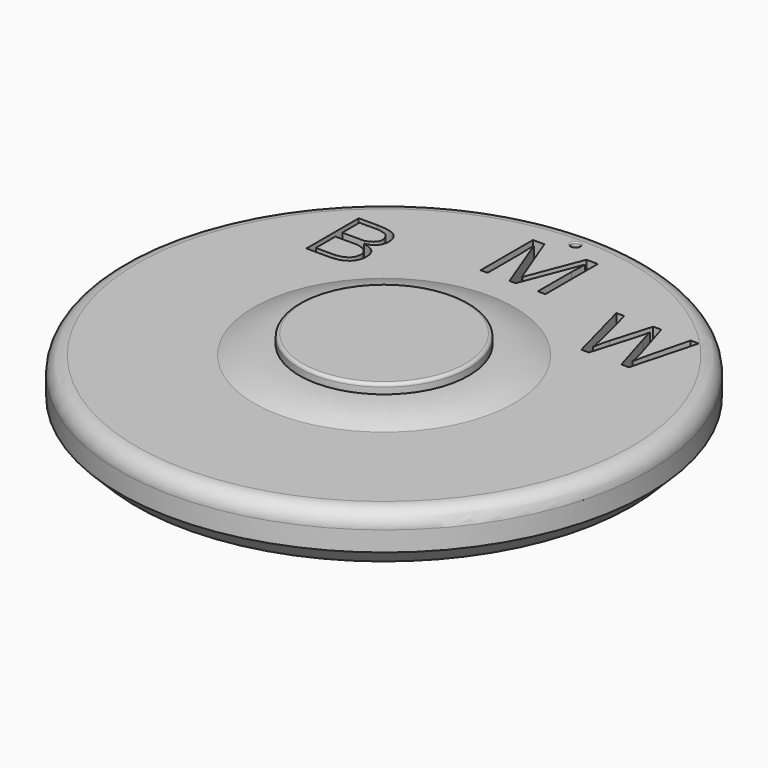
from build123d import *

# Parameters (mm, degrees)
F1_DEPTH   = 18.9
F0_R       = 79.944620776
F2_DEPTH   = 16
F4_R       = 5
F5_SIZE    = 5
F6_DEPTH   = 3
F8_DEPTH   = 2.9
F12_DEPTH  = 16
F13_DEPTH  = 24.3
F15_R      = 0.9656854249
F16_R      = 2.2829721339
F17_DEPTH  = 48.9
F18_R      = 1.3148708501
F18_R_2    = 0.6355346819
F19_DEPTH  = 41.5
F19_FACE_R = 0.6355346819
F20_DEPTH  = 21.5
F21_R      = 0.3379898987


# Not quite as in the source:
# - a fillet or chamfer that OpenCascade refuses, or shapes differently, is made with other operations: its cross-section is extruded or revolved along the edge and cut away or added
# - the program builds the solid bodies; features that only make, move or delete a surface that nothing else refers to are left out


with BuildPart() as f1:
    # F0 (on Top) → F1 (new body)
    with BuildSketch(Plane.XY):
        with BuildLine():
            Line((0, 0), (0, 41.5136932319))
            ThreePointArc((0, 41.5136932319), (-29.3546139964, 29.3546139964), (-41.5136932319, 0))
            Line((-41.5136932319, 0), (0, 0))
        make_face()
        with BuildLine():
            Line((0, 0), (41.5136932319, 0))
            ThreePointArc((41.5136932319, 0), (29.3546139964, 29.3546139964), (0, 41.5136932319))
            Line((0, 41.5136932319), (0, 0))
        make_face()
        with BuildLine():
            ThreePointArc((-41.5136932319, 0), (-29.3546139964, -29.3546139964), (0, -41.5136932319))
            Line((0, -41.5136932319), (0, 0))
            Line((0, 0), (-41.5136932319, 0))
        make_face()
        with BuildLine():
            ThreePointArc((0, -41.5136932319), (29.3546139964, -29.3546139964), (41.5136932319, 0))
            Line((41.5136932319, 0), (0, 0))
            Line((0, 0), (0, -41.5136932319))
        make_face()
    extrude(amount=F1_DEPTH)

    # F0 (on Top) → F2 (join)
    with BuildSketch(Plane.XY):
        Circle(F0_R)
        with BuildLine():
            Line((-48.4910080516, 31.1804282402), (-48.4910080516, 51.0111574069))
            Line((-48.4910080516, 51.0111574069), (-42.8877094405, 51.0111574069))
            add(Edge.make_bspline(
                [(-42.8877094405, 51.0111574069), (-38.9423969405, 51.0111574069), (-37.1780740238, 49.8306018513)],
                knots=[0, 0, 0, 1, 1, 1], degree=2))
            add(Edge.make_bspline(
                [(-37.1780740238, 49.8306018513), (-35.4137511071, 48.6500462958), (-35.4137511071, 46.1023032402)],
                knots=[0, 0, 0, 1, 1, 1], degree=2))
            add(Edge.make_bspline(
                [(-35.4137511071, 46.1023032402), (-35.4137511071, 44.3358101847), (-36.3968240238, 43.1899768513)],
                knots=[0, 0, 0, 1, 1, 1], degree=2))
            add(Edge.make_bspline(
                [(-36.3968240238, 43.1899768513), (-37.3798969405, 42.044143518), (-39.2679177738, 41.7056018513)],
                knots=[0, 0, 0, 1, 1, 1], degree=2))
            Line((-39.2679177738, 41.7056018513), (-39.2679177738, 41.5710532402))
            add(Edge.make_bspline(
                [(-39.2679177738, 41.5710532402), (-34.7496886071, 40.7984837958), (-34.7496886071, 36.8227893513)],
                knots=[0, 0, 0, 1, 1, 1], degree=2))
            add(Edge.make_bspline(
                [(-34.7496886071, 36.8227893513), (-34.7496886071, 34.1665393513), (-36.5465636071, 32.6734837958)],
                knots=[0, 0, 0, 1, 1, 1], degree=2))
            add(Edge.make_bspline(
                [(-36.5465636071, 32.6734837958), (-38.3434386071, 31.1804282402), (-41.5726052738, 31.1804282402)],
                knots=[0, 0, 0, 1, 1, 1], degree=2))
            Line((-41.5726052738, 31.1804282402), (-48.4910080516, 31.1804282402))
        make_face(mode=Mode.SUBTRACT)
        with BuildLine():
            ThreePointArc((0, 41.5136932319), (29.3546139964, 29.3546139964), (41.5136932319, 0))
            ThreePointArc((41.5136932319, 0), (29.3546139964, -29.3546139964), (0, -41.5136932319))
            ThreePointArc((0, -41.5136932319), (-29.3546139964, -29.3546139964), (-41.5136932319, 0))
            ThreePointArc((-41.5136932319, 0), (-29.3546139964, 29.3546139964), (0, 41.5136932319))
        make_face(mode=Mode.SUBTRACT)
        with BuildLine():
            Line((1.2760416667, 48.2220121983), (-0.5815972222, 48.2220121983))
            Line((-0.5815972222, 48.2220121983), (-7.3090277778, 65.8001371983))
            Line((-7.3090277778, 65.8001371983), (-7.4175347222, 65.8001371983))
            add(Edge.make_bspline(
                [(-7.4175347222, 65.8001371983), (-7.2265625, 63.7124635872), (-7.2265625, 60.8348594206)],
                knots=[0, 0, 0, 1, 1, 1], degree=2))
            Line((-7.2265625, 60.8348594206), (-7.2265625, 48.2220121983))
            Line((-7.2265625, 48.2220121983), (-9.3576388889, 48.2220121983))
            Line((-9.3576388889, 48.2220121983), (-9.3576388889, 68.052741365))
            Line((-9.3576388889, 68.052741365), (-5.8854166667, 68.052741365))
            Line((-5.8854166667, 68.052741365), (0.3949652778, 51.6942344206))
            Line((0.3949652778, 51.6942344206), (0.5034722222, 51.6942344206))
            Line((0.5034722222, 51.6942344206), (6.8359375, 68.052741365))
            Line((6.8359375, 68.052741365), (10.2821180556, 68.052741365))
            Line((10.2821180556, 68.052741365), (10.2821180556, 48.2220121983))
            Line((10.2821180556, 48.2220121983), (7.9774305556, 48.2220121983))
            Line((7.9774305556, 48.2220121983), (7.9774305556, 60.9997899761))
            add(Edge.make_bspline(
                [(7.9774305556, 60.9997899761), (7.9774305556, 63.1959705317), (8.1684027778, 65.7740955317)],
                knots=[0, 0, 0, 1, 1, 1], degree=2))
            Line((8.1684027778, 65.7740955317), (8.0598958333, 65.7740955317))
            Line((8.0598958333, 65.7740955317), (1.2760416667, 48.2220121983))
        make_face(mode=Mode.SUBTRACT)
        with BuildLine():
            Line((54.386543, 51.1552815385), (49.0827235555, 31.3245523718))
            Line((49.0827235555, 31.3245523718), (46.8040777222, 31.3245523718))
            Line((46.8040777222, 31.3245523718), (42.8023416111, 44.601462094))
            add(Edge.make_bspline(
                [(42.8023416111, 44.601462094), (42.5158832777, 45.4868787607), (42.1643207777, 46.828024594)],
                knots=[0, 0, 0, 1, 1, 1], degree=2))
            add(Edge.make_bspline(
                [(42.1643207777, 46.828024594), (41.8127582777, 48.1691704274), (41.7997374444, 48.4426079274)],
                knots=[0, 0, 0, 1, 1, 1], degree=2))
            add(Edge.make_bspline(
                [(41.7997374444, 48.4426079274), (41.5002582777, 46.6500732051), (40.8492166111, 44.523337094)],
                knots=[0, 0, 0, 1, 1, 1], degree=2))
            Line((40.8492166111, 44.523337094), (36.9690082777, 31.3245523718))
            Line((36.9690082777, 31.3245523718), (34.6903624444, 31.3245523718))
            Line((34.6903624444, 31.3245523718), (29.4125846666, 51.1552815385))
            Line((29.4125846666, 51.1552815385), (31.8561610555, 51.1552815385))
            Line((31.8561610555, 51.1552815385), (34.9898416111, 38.9070176496))
            add(Edge.make_bspline(
                [(34.9898416111, 38.9070176496), (35.6408832777, 36.3288926496), (35.9403624444, 34.2412190385)],
                knots=[0, 0, 0, 1, 1, 1], degree=2))
            add(Edge.make_bspline(
                [(35.9403624444, 34.2412190385), (36.3049457777, 36.7238579274), (37.0254318888, 39.0979898718)],
                knots=[0, 0, 0, 1, 1, 1], degree=2))
            Line((37.0254318888, 39.0979898718), (40.5757791111, 51.1552815385))
            Line((40.5757791111, 51.1552815385), (43.0193555, 51.1552815385))
            Line((43.0193555, 51.1552815385), (46.7476541111, 38.9894829274))
            add(Edge.make_bspline(
                [(46.7476541111, 38.9894829274), (47.3986957777, 36.8844482051), (47.8457443888, 34.2412190385)],
                knots=[0, 0, 0, 1, 1, 1], degree=2))
            add(Edge.make_bspline(
                [(47.8457443888, 34.2412190385), (48.1061610555, 36.1683023718), (48.8223068888, 38.9330593162)],
                knots=[0, 0, 0, 1, 1, 1], degree=2))
            Line((48.8223068888, 38.9330593162), (51.9429666111, 51.1552815385))
            Line((51.9429666111, 51.1552815385), (54.386543, 51.1552815385))
        make_face(mode=Mode.SUBTRACT)
    extrude(amount=F2_DEPTH)

    # F3: chamfer of 5 on 1 edges, made by hand


with BuildPart() as f3_tool2:
    # F3_s3 → F3_t4 (revolve)
    with BuildSketch(Plane.YZ):
        Polygon((-41.5136932319, 13.9), (-36.5136932319, 18.9), (-41.5136932319, 18.9), align=None)
    revolve(axis=Axis((0, 0, 18.9), (0, 0, 1)))

    split(bisect_by=Plane.XY.offset(16), keep=Keep.TOP)


with BuildPart() as f1_1:
    add(f1.part)

    # F3_t1: cut F3_tool2
    add(f3_tool2.part, mode=Mode.SUBTRACT)

    # F4
    f4_edges = [f1_1.edges().sort_by_distance(p)[0] for p in [
        (-79.944621, 0, 16),
    ]]
    fillet(f4_edges, radius=F4_R)

    # F5
    f5_edges = [f1_1.edges().sort_by_distance(p)[0] for p in [
        (-79.944621, 0, 0),
    ]]
    chamfer(f5_edges, length=F5_SIZE)

    # F6 (add): a face of the model
    f6_faces = [f1_1.faces().sort_by_distance(p)[0] for p in [
        (0, 0, 18.9),
    ]]
    extrude(f6_faces, amount=-F6_DEPTH)

    # F7: fillet of radius 33.9837993167 on 1 edges, made by hand

    # F7_s1 → F7_t2 (revolve, cut)
    with BuildSketch(Plane.YZ):
        with BuildLine():
            ThreePointArc((-39.4136932319, 16), (-32.6967485164, 18.1670970169), (-25.677025658, 18.9))
            Line((-25.677025658, 18.9), (-36.5136932319, 18.9))
            Line((-36.5136932319, 18.9), (-39.4136932319, 16))
        make_face()
    revolve(axis=Axis((0, 0, 18.9), (0, 0, 1)), mode=Mode.SUBTRACT)

    # F8 (add): a face of the model
    f8_faces = [f1_1.faces().sort_by_distance(p)[0] for p in [
        (0, 0, 18.9),
    ]]
    extrude(f8_faces, amount=F8_DEPTH)

    # F13 (add): a face of the model
    f13_faces = [f1_1.faces().sort_by_distance(p)[0] for p in [
        (0, 0, 21.8),
    ]]
    extrude(f13_faces, amount=-F13_DEPTH)

    # F15
    f15_edges = [f1_1.edges().sort_by_distance(p)[0] for p in [
        (0, 25.677026, 21.8),
    ]]
    fillet(f15_edges, radius=F15_R)

    # F16 (on Top) → F17 (cut)
    with BuildSketch(Plane.XY):
        with Locations((0, 71.3628157973)):
            Circle(F16_R)
    extrude(amount=-F17_DEPTH, mode=Mode.SUBTRACT)

    # F18 (on Top) → F19 (cut)
    with BuildSketch(Plane.XY):
        with Locations((0, 72.516053915)):
            Circle(F18_R)
        with Locations((0, 72.516053915)):
            Circle(F18_R_2, mode=Mode.SUBTRACT)
    extrude(amount=F19_DEPTH, mode=Mode.SUBTRACT)

    # F18 (on Top) + F19_face (on face) → F20 (cut)
    with BuildSketch(Plane.XY):
        with Locations((0, 72.516053915)):
            Circle(F18_R)
        with Locations((0, 72.516053915)):
            Circle(F18_R_2, mode=Mode.SUBTRACT)
    with BuildSketch(Plane(origin=(0, 72.516053915, 16), x_dir=(1, 0, 0), z_dir=(0, 0, 1))):
        Circle(F19_FACE_R)
    extrude(amount=-F20_DEPTH, mode=Mode.SUBTRACT)

    # F21
    f21_edges = [f1_1.edges().sort_by_distance(p)[0] for p in [
        (-1.314871, 72.516054, 16),
    ]]
    fillet(f21_edges, radius=F21_R)


with BuildPart() as f12:
    # F11 (on Top) → F12 (new body)
    with BuildSketch(Plane.XY):
        with BuildLine():
            Line((-41.1170236766, 49.3229441345), (-46.9156317413, 49.3229441345))
            Line((-46.9156317413, 49.3229441345), (-46.9156317413, 42.8233034909))
            Line((-46.9156317413, 42.8233034909), (-44.3502888083, 42.8233034909))
            Line((-44.3502888083, 42.8233034909), (-40.2086749673, 42.8233034909))
            add(Edge.make_bspline(
                [(-41.1170236766, 49.3229441345), (-39.204246299, 48.9134589045), (-37.7507729109, 48.8444333294), (-36.1566804349, 44.0774895251), (-40.2086749673, 42.8233034909)],
                knots=[0, 0, 0, 0, 0.4415569588, 1, 1, 1, 1], degree=3))
        make_face()
    extrude(amount=F12_DEPTH)


with BuildPart() as f12b:
    # F11 (on Top) → F12, piece 2 (new body)
    with BuildSketch(Plane.XY):
        with BuildLine():
            Line((-46.9156317413, 40.2184464037), (-46.9156317413, 32.8139699996))
            Line((-46.9156317413, 32.8139699996), (-41.1170236766, 32.8139699996))
            add(Edge.make_bspline(
                [(-41.1170236766, 32.8139699996), (-37.7967730165, 33.1756919622), (-35.7796114313, 35.9142584701), (-36.8320122361, 39.5431146026), (-40.2086749673, 40.2184464037)],
                knots=[0, 0, 0, 0, 0.5046489381, 1, 1, 1, 1], degree=3))
            Line((-40.2086749673, 40.2184464037), (-44.3502888083, 40.2184464037))
            Line((-44.3502888083, 40.2184464037), (-46.9156317413, 40.2184464037))
        make_face()
    extrude(amount=F12_DEPTH)


solid = Compound([f1_1.part, f12.part, f12b.part])
